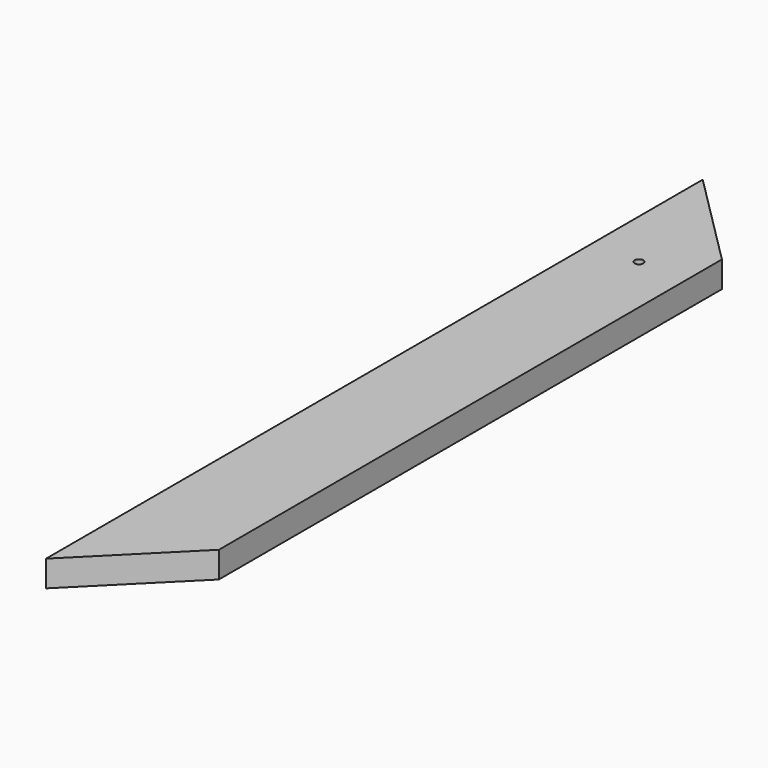
from build123d import *

# Parameters (mm, degrees)
F0_W      = 139.7
F0_H      = 38.1
F1_DEPTH  = 1828.8
F3_W      = 331.3202857971
F3_H      = 260.5838701129
F4_DEPTH  = 101.6
F7_W      = 1553.4552037716
F7_H      = 1155.3529500961
F8_DEPTH  = 762
F9_R      = 6.35
F10_DEPTH = 38.101


# Not quite as in the source:
# - a feature names something its author has since deleted; it is built from what else it names


with BuildPart() as f1:
    # F0 (on Front) → F1 (new body)
    with BuildSketch(Plane.XZ):
        with Locations((69.85, 19.05)):
            Rectangle(F0_W, F0_H)
    extrude(amount=F1_DEPTH)

    # F3 (on face) → F4 (cut)
    with BuildSketch(Plane(origin=(984.25, -984.25, 0), x_dir=(-0.7071067812, -0.7071067812, 0), z_dir=(-0.7071067812, 0.7071067812, 0))):
        with Locations((1222.6701974869, 7.0506222546)):
            Rectangle(F3_W, F3_H)
    extrude(amount=F4_DEPTH, mode=Mode.SUBTRACT)

    # F7 (on face) → F8 (cut)
    with BuildSketch(Plane(origin=(-315.2209189803, -315.2209189803, 0), x_dir=(0.7071067812, -0.7071067812, 0), z_dir=(-0.7071067812, -0.7071067812, 0))):
        with Locations((614.4417077303, -181.5140247345)):
            Rectangle(F7_W, F7_H)
    extrude(amount=-F8_DEPTH, mode=Mode.SUBTRACT)

    # F9 (on face) → F10 (cut, through all)
    with BuildSketch(Plane.XY.offset(38.1)):
        with Locations((69.85, -833.6418379607)):
            Circle(F9_R)
    extrude(amount=-F10_DEPTH, mode=Mode.SUBTRACT)


solid = f1.part
